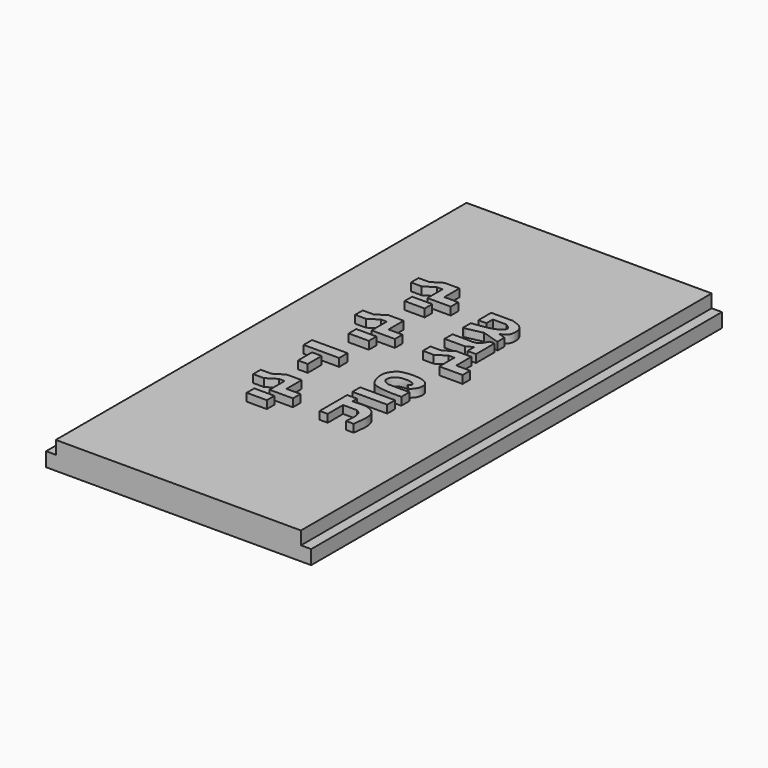
from build123d import *

# Parameters (mm, degrees)
F0_W     = 46.8
F0_H     = 2.5
F1_DEPTH = 49
F2_W     = 7.5
F2_H     = 1
F5_W     = 2.0469846204
F5_H     = 1.8061620649
F5_W_2   = 6.6439194979
F5_H_2   = 1.8455331939
F5_W_3   = 3.8363870533
F5_H_3   = 1.8061622977
F5_W_4   = 1.0836967267
F5_W_5   = 6.7777763455
F5_H_4   = 2
F5_W_6   = 1.8455331939
F5_H_5   = 3.3219597489
F6_DEPTH = 1.5


# Not quite as in the source:
# - a fillet or chamfer that OpenCascade refuses, or shapes differently, is made with other operations: its cross-section is extruded or revolved along the edge and cut away or added


with BuildPart() as f1:
    # F0 (on Front) → F1 (new body, symmetric)
    with BuildSketch(Plane.XZ):
        Polygon((25.3, -1.35), (25.3, 1.35), (23.3460554371, 1.35), (-23.4539445629, 1.35), (-25.3, 1.35), (-25.3, -1.35), align=None)
        with Locations((-0.0539445629, 2.6)):
            Rectangle(F0_W, F0_H)
    extrude(amount=F1_DEPTH, both=True)

    # F2 (on Front) → F3 (revolve, cut)
    with BuildSketch(Plane.XZ):
        with Locations((3.75, -0.85)):
            Rectangle(F2_W, F2_H)
    revolve(axis=Axis((0, 0, -0.85), (0, 0, -1)), mode=Mode.SUBTRACT)

    # F4: fillet of radius 5 on 1 edges, made by hand

    # F4_s1 → F4_t2 (revolve)
    with BuildSketch(Plane.XZ):
        with BuildLine():
            ThreePointArc((7.5, -1.35), (6.0811388301, -0.6065835097), (4.5, -0.35))
            Line((4.5, -0.35), (7.5, -0.35))
            Line((7.5, -0.35), (7.5, -1.35))
        make_face()
    revolve(axis=Axis((0, 0, -0.35), (0, 0, -1)))

    # F5 (on face) → F6 (join)
    with BuildSketch(Plane.XY.offset(3.85)):
        with BuildLine():
            Line((4.9241716042, 19.8006471619), (7.5009630335, 19.8006471619))
            add(Edge.make_bspline(
                [(7.5009630335, 19.8006471619), (7.9785124596, 19.5075781217), (8.9543671976, 18.9087022865), (7.3816458851, 17.3276064651), (4.7697273037, 17.0174018652), (3.1129348501, 16.8206328526)],
                knots=[0, 0, 0, 0, 0.2595051335, 0.5302892228, 1, 1, 1, 1], degree=3))
            Line((3.1129348501, 16.8206328526), (3.1129348501, 14.9474805221))
            Line((3.1129348501, 14.9474805221), (3.4767354373, 14.9474805221))
            add(Edge.make_bspline(
                [(3.4767354373, 14.9474805221), (4.5253869977, 15.1745288943), (5.5740385582, 15.4015772666), (6.6226901187, 15.6286256388)],
                knots=[0, 0, 0, 0, 3.2188490998, 3.2188490998, 3.2188490998, 3.2188490998], degree=3))
            Line((6.6226901187, 15.6286256388), (9.9595930205, 14.6069070324))
            Line((9.9595930205, 14.6069070324), (9.9595930205, 16.3097716868))
            Line((9.9595930205, 16.3097716868), (8.527294053, 16.7483240055))
            add(Edge.make_bspline(
                [(8.527294053, 16.7483240055), (9.0505266558, 16.9185557016), (10.2287332466, 17.301880642), (10.2116405832, 20.5168892904), (8.4127583201, 21.0586346497), (7.5009630335, 21.3332278654)],
                knots=[0, 0, 0, 0, 0.2826109345, 0.6363786658, 1, 1, 1, 1], degree=3))
            Line((7.5009630335, 21.3332278654), (3.3915922977, 21.3332278654))
            Line((3.3915922977, 21.3332278654), (3.3915922977, 18.2680701837))
            Line((3.3915922977, 18.2680701837), (4.9241716042, 18.2680701837))
            Line((4.9241716042, 18.2680701837), (4.9241716042, 19.8006471619))
        make_face()
        with BuildLine():
            Line((5.1796017215, 12.3080369085), (3.2213055529, 12.3080369085))
            Line((3.2213055529, 12.3080369085), (3.2213055529, 10.434884578))
            Line((3.2213055529, 10.434884578), (3.987595439, 10.434884578))
            add(Edge.make_bspline(
                [(7.0864924639, 10.434884578), (6.6226901187, 10.434884578), (5.6548767314, 10.434884578), (4.5585386607, 10.434884578), (3.987595439, 10.434884578)],
                knots=[0, 0, 0, 0, 0.4792270404, 1, 1, 1, 1], degree=3))
            add(Edge.make_bspline(
                [(7.0864924639, 10.434884578), (7.5009630335, 10.6619332607), (7.915433603, 10.8889819433), (8.3299041726, 11.116030626)],
                knots=[0, 0, 0, 0, 1.4177561906, 1.4177561906, 1.4177561906, 1.4177561906], degree=3))
            Line((8.3299041726, 11.116030626), (8.3299041726, 12.7337537706))
            add(Edge.make_bspline(
                [(5.1796017215, 12.3080369085), (5.4034691903, 12.3161910935), (5.946247887, 12.3359613528), (7.5456770883, 12.1555160266), (8.0916682054, 12.558094155), (8.3299041726, 12.7337537706)],
                knots=[0, 0, 0, 0, 0.2835019002, 0.6873655771, 1, 1, 1, 1], degree=3))
        make_face()
        with BuildLine():
            add(Edge.make_bspline(
                [(8.3299041726, 12.7337537706), (8.5748998169, 13.1310888877), (8.8198954612, 13.5284240047), (9.0648911056, 13.9257591218)],
                knots=[0, 0, 0, 0, 1.4003865712, 1.4003865712, 1.4003865712, 1.4003865712], degree=3))
            Line((8.3299041726, 12.7337537706), (8.3299041726, 11.116030626))
            Line((8.3299041726, 11.116030626), (8.3299041726, 9.4983074814))
            Line((8.3299041726, 9.4983074814), (9.0648911056, 9.4983074814))
            Line((9.0648911056, 9.4983074814), (9.9595930205, 9.4983074814))
            Line((9.9595930205, 9.4983074814), (9.9595930205, 13.9257591218))
            Line((9.9595930205, 13.9257591218), (9.0648911056, 13.9257591218))
        make_face()
        Polygon((8.1701891906, 8.3958084671), (7.0864924639, 8.3958084671), (5.1599194705, 7.1917017432), (5.1599194705, 5.3855396783), (7.0864924639, 6.5896464022), (8.1701891906, 6.5896464022), align=None)
        with Locations((4.1364271603, 6.2886207107)):
            Rectangle(F5_W, F5_H)
        Polygon((9.9595930205, 8.3958084671), (8.1701891906, 8.3958084671), (8.1701891906, 6.5896464022), (8.1701891906, 4.7834843373), (9.9595930205, 4.7834843373), align=None)
        Polygon((12.62538982, 4.7834843373), (9.9595930205, 4.7834843373), (8.1701891906, 4.7834843373), (8.1701891906, 2.9773220395), (12.62538982, 2.9773220395), align=None)
        with BuildLine():
            Line((8.1941955723, -4.5991633087), (9.157482069, -5.5624498054))
            add(Edge.make_bspline(
                [(9.157482069, -5.5624498054), (9.5487792454, -5.1790893624), (10.3709560961, -4.3735888355), (10.1809148183, -1.5911495575), (5.2901881268, -1.6214904462), (3.9387879664, -2.4019349259), (2.8327143669, -4.2152866088), (3.4405306211, -6.4549250287), (4.2493320025, -7.9388718891), (8.0091011439, -8.2673740434), (9.3225151381, -8.2281395815), (9.8799471743, -8.2114879042)],
                knots=[0, 0, 0, 0, 0.0955972377, 0.2008648172, 0.3547140558, 0.449658727, 0.5522106806, 0.6629402054, 0.7557007662, 0.8963158456, 1, 1, 1, 1], degree=3))
            Line((9.8799471743, -8.2114879042), (9.8799471743, -6.2849144451))
            Line((9.8799471743, -6.2849144451), (9.639125783, -6.2849144451))
            Line((9.639125783, -6.2849144451), (5.7859793305, -6.2849144451))
            add(Edge.make_bspline(
                [(5.7859793305, -6.2849144451), (5.3373815573, -6.0824238319), (4.5029895973, -5.7057912452), (4.6151304787, -4.5054927526), (5.5221677114, -3.357555761), (8.2143823017, -3.3336799886), (8.8829973904, -4.2841414137), (8.4141443171, -4.4985702665), (8.1941955723, -4.5991633087)],
                knots=[0, 0, 0, 0, 0.1746613826, 0.3248702113, 0.5034996406, 0.7468657523, 0.8812494506, 1, 1, 1, 1], degree=3))
        make_face()
        with Locations((6.4990330953, -10.5825328623)):
            Rectangle(F5_W_2, F5_H_2)
        with BuildLine():
            Line((5.094458349, -12.8092374653), (3.2213055529, -12.8092374653))
            Line((3.2213055529, -12.8092374653), (3.2213055529, -19.3652724847))
            Line((3.2213055529, -19.3652724847), (4.753885325, -19.3652724847))
            Line((4.753885325, -19.3652724847), (4.753885325, -15.7041111961))
            Line((4.753885325, -15.7041111961), (7.393327076, -15.7041111961))
            add(Edge.make_bspline(
                [(7.393327076, -15.7041111961), (7.7280745564, -15.8906025071), (8.6028551514, -16.3779518959), (8.4340893146, -18.2776591394), (8.3299041726, -19.4504158571)],
                knots=[0, 0, 0, 0, 0.3826645017, 1, 1, 1, 1], degree=3))
            Line((8.3299041726, -19.4504158571), (9.777339641, -19.4504158571))
            add(Edge.make_bspline(
                [(9.777339641, -19.4504158571), (9.916282957, -18.4574178062), (10.1622140126, -16.6998013476), (9.7862090494, -14.9229979542), (8.1515194, -13.6961261057), (6.2020376655, -13.8364032587), (5.094458349, -13.9161003754)],
                knots=[0, 0, 0, 0, 0.2773941316, 0.4909903808, 0.7108110755, 1, 1, 1, 1], degree=3))
            Line((5.094458349, -13.9161003754), (5.094458349, -12.8092374653))
        make_face()
        Polygon((-8.0897600321, 22.7236154125), (-7.0060633053, 22.7236154125), (-7.0060633053, 24.5297774774), (-8.0897600321, 24.5297774774), (-10.0163330255, 23.3256707535), (-12.0633176458, 23.3256707535), (-12.0633176458, 21.5195086886), (-10.0163330255, 21.5195086886), align=None)
        Polygon((-7.0060633053, 20.9174533476), (-5.2166594755, 20.9174533476), (-5.2166594755, 24.5297774774), (-7.0060633053, 24.5297774774), (-7.0060633053, 22.7236154125), align=None)
        Polygon((-7.0060633053, 19.1112910499), (-2.550862676, 19.1112910499), (-2.550862676, 20.9174533476), (-5.2166594755, 20.9174533476), (-7.0060633053, 20.9174533476), align=None)
        with Locations((-7.1348530021, 17.1245136399)):
            Rectangle(F5_W_3, F5_H_3)
        Polygon((-9.9878371693, 8.1643839367), (-8.0612641759, 9.3684906606), (-8.0612641759, 11.1746527255), (-9.9878371693, 9.9705460016), (-12.0348217897, 9.9705460016), (-12.0348217897, 8.1643839367), align=None)
        with Locations((-7.5194158126, 10.271571693)):
            Rectangle(F5_W_4, F5_H)
        Polygon((-6.9775674492, 9.3684906606), (-6.9775674492, 7.5623285957), (-5.1881636194, 7.5623285957), (-5.1881636194, 11.1746527255), (-6.9775674492, 11.1746527255), align=None)
        Polygon((-6.9775674492, 5.7561662979), (-2.5223668199, 5.7561662979), (-2.5223668199, 7.5623285957), (-5.1881636194, 7.5623285957), (-6.9775674492, 7.5623285957), align=None)
        with Locations((-7.106357146, 3.769388888)):
            Rectangle(F5_W_3, F5_H_3)
        with Locations((-8.5770517921, -3.2183615263)):
            Rectangle(F5_W_5, F5_H_4)
        with Locations((-8.560137578, -6.9900213829)):
            Rectangle(F5_W_6, F5_H_5)
        Polygon((-7.969349802, -15.0853700369), (-6.8856530753, -15.0853700369), (-6.8856530753, -13.279207972), (-7.969349802, -13.279207972), (-9.8959227954, -14.4833146959), (-11.9429074158, -14.4833146959), (-11.9429074158, -16.2894767608), (-9.8959227954, -16.2894767608), align=None)
        Polygon((-6.8856530753, -15.0853700369), (-6.8856530753, -16.8915321018), (-5.0962492455, -16.8915321018), (-5.0962492455, -13.279207972), (-6.8856530753, -13.279207972), align=None)
        Polygon((-6.8856530753, -18.6976943995), (-2.430452446, -18.6976943995), (-2.430452446, -16.8915321018), (-5.0962492455, -16.8915321018), (-6.8856530753, -16.8915321018), align=None)
        with Locations((-7.0144427721, -20.6844718094)):
            Rectangle(F5_W_3, F5_H_3)
    extrude(amount=F6_DEPTH)


solid = f1.part
